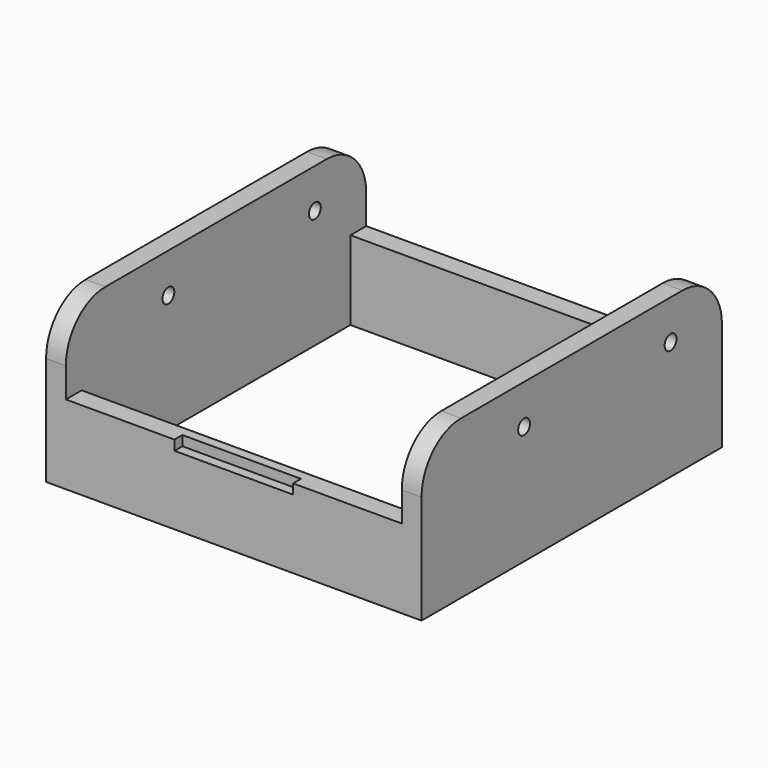
from build123d import *

# Parameters (mm, degrees)
F0_W          = 38
F0_H          = 38
F0_W_2        = 34
F0_H_2        = 34
F1_DEPTH      = 8
F3_DEPTH      = 1
F5_DEPTH      = 8
F6_R          = 0.75
F7_DEPTH      = 50.7
F7_DEPTH_BACK = 53.4
F8_R          = 5


with BuildPart() as f1:
    # F0 (on Top) → F1 (new body)
    with BuildSketch(Plane.XY):
        with Locations((19, 19)):
            Rectangle(F0_W, F0_H)
        with Locations((19, 19)):
            Rectangle(F0_W_2, F0_H_2, mode=Mode.SUBTRACT)
    extrude(amount=F1_DEPTH)

    # F2 (on face) → F3 (cut)
    with BuildSketch(Plane.XY.offset(8)):
        Polygon((13, 0), (19, 0), (25, 0), (25, 1), (19, 1), (13, 1), align=None)
    extrude(amount=-F3_DEPTH, mode=Mode.SUBTRACT)

    # F4 (on face) → F5 (join)
    with BuildSketch(Plane.XY.offset(8)):
        Polygon((0, 38), (0, 0), (2, 0), (2, 2), (2, 36), (2, 38), align=None)
        Polygon((38, 38), (36, 38), (36, 36), (36, 2), (36, 0), (38, 0), align=None)
    extrude(amount=F5_DEPTH)

    # F6 (on face) → F7 (cut, two sides)
    with BuildSketch(Plane(origin=(36, 0, 0), x_dir=(0, -1, 0), z_dir=(-1, 0, 0))) as f7_sk:
        with Locations((-31.5038709193, 12)):
            Circle(F6_R)
        with Locations((-12.9723072276, 12)):
            Circle(F6_R)
    extrude(amount=-F7_DEPTH, mode=Mode.SUBTRACT)
    extrude(f7_sk.sketch, amount=F7_DEPTH_BACK, mode=Mode.SUBTRACT)

    # F8
    f8_edges = [f1.edges().sort_by_distance(p)[0] for p in [
        (1, 0, 16),
        (37, 0, 16),
        (37, 38, 16),
        (1, 38, 16),
    ]]
    fillet(f8_edges, radius=F8_R)


solid = f1.part
